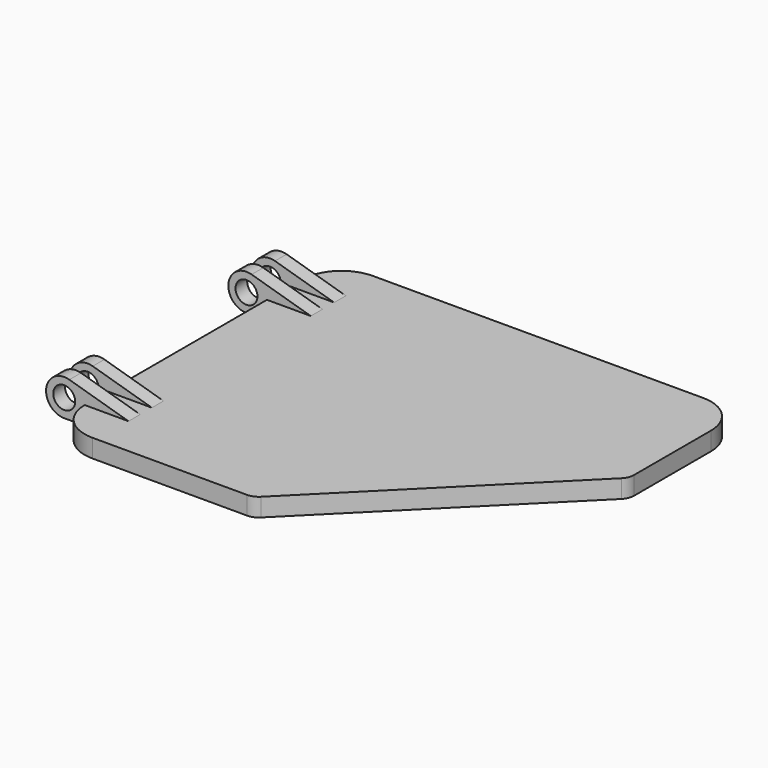
from build123d import *

# Parameters (mm, degrees)
F1_DEPTH = 1.25
F2_W     = 6
F2_H     = 1
F3_DEPTH = 2.5
F4_R     = 0.75
F5_DEPTH = 75


# Not quite as in the source:
# - a feature names something its author has since deleted; it is built from what else it names


with BuildPart() as f1:
    # F0 (on Top) → F1 (new body)
    with BuildSketch(Plane.XY):
        with BuildLine():
            ThreePointArc((-7.984982332, 15.2434693582), (-9.8941706412, 14.4526576674), (-10.684982332, 12.5434693582))
            Line((-10.684982332, 12.5434693582), (-10.684982332, -6.0565306418))
            ThreePointArc((-10.684982332, -6.0565306418), (-9.8941706412, -7.965718951), (-7.984982332, -8.7565306418))
            Line((-7.984982332, -8.7565306418), (2.6008041056, -8.7565306418))
            ThreePointArc((2.6008041056, -8.7565306418), (2.983487538, -8.6804101743), (3.3079108868, -8.463637423))
            Line((3.3079108868, -8.463637423), (17.0221244492, 5.2505761394))
            ThreePointArc((17.0221244492, 5.2505761394), (17.2388972005, 5.5749994882), (17.315017668, 5.9576829206))
            Line((17.315017668, 5.9576829206), (17.315017668, 12.5434693582))
            ThreePointArc((17.315017668, 12.5434693582), (16.5242059772, 14.4526576674), (14.615017668, 15.2434693582))
            Line((14.615017668, 15.2434693582), (-7.984982332, 15.2434693582))
        make_face()
    extrude(amount=F1_DEPTH)

    # F2 (on face) → F3 (join, symmetric)
    with BuildSketch(Plane.XY.offset(1.25)):
        Polygon((-7.684982332, 12.5434693582), (-10.684982332, 12.5434693582), (-13.684982332, 12.5434693582), (-13.684982332, 11.5434693582), (-10.684982332, 11.5434693582), (-7.684982332, 11.5434693582), align=None)
        with Locations((-10.684982332, 10.0434693582)):
            Rectangle(F2_W, F2_H)
        Polygon((-13.684982332, -6.0565306418), (-10.684982332, -6.0565306418), (-7.684982332, -6.0565306418), (-7.684982332, -5.0565306418), (-10.684982332, -5.0565306418), (-13.684982332, -5.0565306418), align=None)
        with Locations((-10.684982332, -3.5565306418)):
            Rectangle(F2_W, F2_H)
    extrude(amount=F3_DEPTH, both=True)

    # F4 (on face) → F5 (cut)
    with BuildSketch(Plane.XZ.offset(6.0565306418)):
        with BuildLine():
            Line((-11.7352277888, 2.4365543881), (-7.684982332, 1.25))
            Line((-7.684982332, 1.25), (-7.684982332, 3.75))
            Line((-7.684982332, 3.75), (-13.684982332, 3.75))
            Line((-13.684982332, 3.75), (-13.684982332, -1.25))
            Line((-13.684982332, -1.25), (-7.684982332, -1.25))
            Line((-7.684982332, -1.25), (-7.684982332, 0))
            Line((-7.684982332, 0), (-10.684982332, 0))
            Line((-10.684982332, 0), (-12.0847867802, 0))
            ThreePointArc((-12.0847867802, 0), (-13.3155374428, 1.4199208375), (-11.7352277888, 2.4365543881))
        make_face()
        with Locations((-12.0847867802, 1.2433518423)):
            Circle(F4_R)
    extrude(amount=-F5_DEPTH, mode=Mode.SUBTRACT)


solid = f1.part
